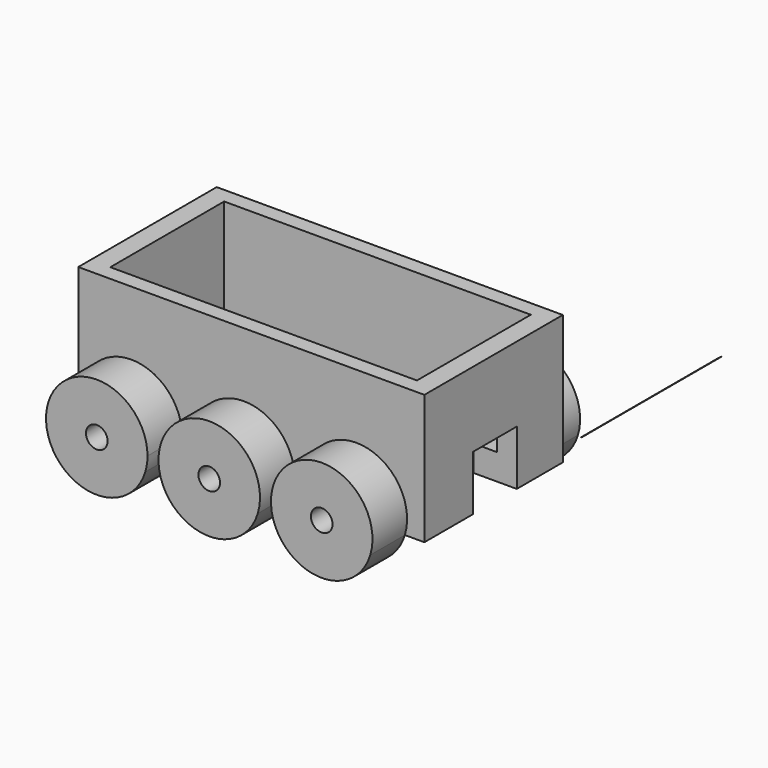
from build123d import *

# Parameters (mm, degrees)
F1_DEPTH  = 25.4
F2_R      = 3.175
F3_DEPTH  = 12.7
F5_W      = 90.0154933333
F5_H      = 41.784722358
F6_DEPTH  = 30.48
F7_W      = 16.129
F7_H      = 16.1236341841
F8_DEPTH  = 12.7
F9_DEPTH  = 25.4
F10_DEPTH = 101.6
F11_DEPTH = 12.7


# Not quite as in the source:
# - a feature names something its author has since deleted; it is built from what else it names


with BuildPart() as f1:
    # F0 (on Front) → F1 (new body, symmetric)
    with BuildSketch(Plane.XZ):
        with BuildLine():
            Line((97.5067541003, 23.5131774098), (96.6568392289, 22.9320458975))
            ThreePointArc((96.6568392289, 22.9320458975), (97.1017650033, 23.1934076134), (97.5067541003, 23.5131774098))
        make_face()
    extrude(amount=F1_DEPTH, both=True)


with BuildPart() as f1b:
    # F0 (on Front) → F1, piece 2 (new body, symmetric)
    with BuildSketch(Plane.XZ):
        Polygon((-50.8, -19.05), (50.8, -19.05), (50.8, -8.4226876497), (50.8, 0), (50.8, 19.05), (-50.8, 19.05), align=None)
    extrude(amount=F1_DEPTH, both=True)



with BuildPart() as f3:
    # F2 (on face) → F3 (new body)
    with BuildSketch(Plane.XZ.offset(25.4)):
        with BuildLine():
            Line((45.0727086193, -19.05), (16.5752838461, -19.05))
            ThreePointArc((16.5752838461, -19.05), (30.8239962327, -29.6026037673), (45.0727086193, -19.05))
        make_face()
        with BuildLine():
            ThreePointArc((45.72, -14.7066), (28.628312416, 0.0266922598), (16.5752838461, -19.05))
            Line((16.5752838461, -19.05), (45.0727086193, -19.05))
            ThreePointArc((45.0727086193, -19.05), (45.5572884925, -16.9022838167), (45.72, -14.7066))
        make_face()
        with Locations((30.8239962327, -14.7066)):
            Circle(F2_R, mode=Mode.SUBTRACT)
    extrude(amount=F3_DEPTH)


with BuildPart() as f3b:
    # F2 (on face) → F3, piece 2 (new body)
    with BuildSketch(Plane.XZ.offset(25.4)):
        with BuildLine():
            ThreePointArc((12.7, -14.7066), (-4.391687584, 0.0266922598), (-16.4447161539, -19.05))
            Line((-16.4447161539, -19.05), (12.0527086193, -19.05))
            ThreePointArc((12.0527086193, -19.05), (12.5372884925, -16.9022838167), (12.7, -14.7066))
        make_face()
        with Locations((-2.1960037673, -14.7066)):
            Circle(F2_R, mode=Mode.SUBTRACT)
        with BuildLine():
            Line((12.0527086193, -19.05), (-16.4447161539, -19.05))
            ThreePointArc((-16.4447161539, -19.05), (-2.1960037673, -29.6026037673), (12.0527086193, -19.05))
        make_face()
    extrude(amount=F3_DEPTH)


with BuildPart() as f3c:
    # F2 (on face) → F3, piece 3 (new body)
    with BuildSketch(Plane.XZ.offset(25.4)):
        with BuildLine():
            ThreePointArc((-20.9686848198, -19.05), (-20.4830637187, -16.9000772846), (-20.32, -14.7020313889))
            ThreePointArc((-20.32, -14.7020313889), (-37.414049663, 0.0309086597), (-49.4633227148, -19.05))
            Line((-49.4633227148, -19.05), (-20.9686848198, -19.05))
        make_face()
        with Locations((-35.2160037673, -14.7020313889)):
            Circle(F2_R, mode=Mode.SUBTRACT)
        with BuildLine():
            Line((-20.9686848198, -19.05), (-49.4633227148, -19.05))
            ThreePointArc((-49.4633227148, -19.05), (-35.2160037673, -29.5980351562), (-20.9686848198, -19.05))
        make_face()
    extrude(amount=F3_DEPTH)


with BuildPart() as f1b_1:
    add(f1b.part)

    add(f3.part)  # F4 merges F3

    add(f3b.part)  # F4 merges F3b

    add(f3c.part)  # F4 merges F3c
    # F4: F3, F3b, F3c across plane
    add(f3.part.mirror(Plane.XZ))
    add(f3b.part.mirror(Plane.XZ))
    add(f3c.part.mirror(Plane.XZ))

    # F5 (on face) → F6 (cut)
    with BuildSketch(Plane.XY.offset(19.05)):
        Rectangle(F5_W, F5_H)
    extrude(amount=-F6_DEPTH, mode=Mode.SUBTRACT)

    # F2 (on face) → F9 (cut)
    with BuildSketch(Plane.XZ.offset(25.4)):
        with Locations((-35.2160037673, -14.7020313889)):
            Circle(F2_R)
        with Locations((-2.1960037673, -14.7066)):
            Circle(F2_R)
        with Locations((30.8239962327, -14.7066)):
            Circle(F2_R)
    extrude(amount=-F9_DEPTH, mode=Mode.SUBTRACT)

    # F2 (on face) → F10 (cut)
    with BuildSketch(Plane.XZ.offset(25.4)):
        with Locations((-2.1960037673, -14.7066)):
            Circle(F2_R)
        with Locations((-35.2160037673, -14.7020313889)):
            Circle(F2_R)
        with Locations((30.8239962327, -14.7066)):
            Circle(F2_R)
    extrude(amount=-F10_DEPTH, mode=Mode.SUBTRACT)


with BuildPart() as f8:
    # F7 (on face) → F8 (new body)
    with BuildSketch(Plane.YZ.offset(50.8)):
        with Locations((0.4445, -10.988182908)):
            Rectangle(F7_W, F7_H)
    extrude(amount=-F8_DEPTH)


with BuildPart() as f11_tool:
    # F7 (on face) → F11 (new body)
    with BuildSketch(Plane.YZ.offset(50.8)):
        with Locations((0.4445, -10.988182908)):
            Rectangle(F7_W, F7_H)
    extrude(amount=-F11_DEPTH)


with BuildPart() as f1b_2:
    add(f1b_1.part)

    # F11: cut by f11_tool
    add(f11_tool.part, mode=Mode.SUBTRACT)


with BuildPart() as f8_1:
    add(f8.part)

    # F11: cut by f11_tool
    add(f11_tool.part, mode=Mode.SUBTRACT)


solid = Compound([f1.part, f1b_2.part])
